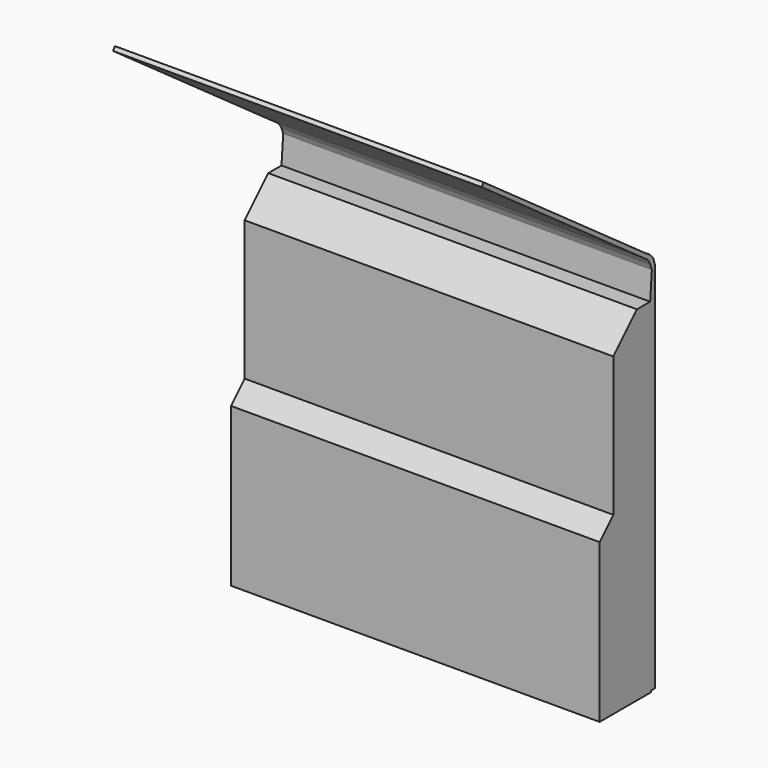
from build123d import *

# Parameters (mm, degrees)
F1_DEPTH    = 31.75
F2_T1_DEPTH = 89.6282991577
F2_T6_DEPTH = 89.6282991577
F4_DEPTH    = 31.75


# Not quite as in the source:
# - a fillet or chamfer that OpenCascade refuses, or shapes differently, is made with other operations: its cross-section is extruded or revolved along the edge and cut away or added


with BuildPart() as f1:
    # F0 (on Right) → F1 (new body, symmetric)
    with BuildSketch(Plane.YZ):
        Polygon((5.5137062445, 29.6514853835), (-2.5730628986, 29.6514853835), (-2.5730628986, 2.6955895592), (-5.5137062445, 2.6955895592), (-5.5137062445, -29.6514853835), (5.5137062445, -29.6514853835), align=None)
    extrude(amount=F1_DEPTH, both=True)

    # F2: chamfer of 5.08 on 2 edges, made by hand

    # F2_s2 → F2_t1 (cut)
    with BuildSketch(Plane.YZ.offset(-44.8141495789)):
        Polygon((2.5069371014, 29.6514853835), (-2.5730628986, 24.5714853835), (-2.5730628986, 29.6514853835), align=None)
    extrude(amount=F2_T1_DEPTH, mode=Mode.SUBTRACT)


with BuildPart() as f2_tool4:
    # F2_s5 → F2_t6 (new body)
    with BuildSketch(Plane.YZ.offset(-44.8141495789)):
        Polygon((-5.5137062445, -2.3844104408), (-0.4337062445, 2.6955895592), (-5.5137062445, 2.6955895592), align=None)
    extrude(amount=F2_T6_DEPTH)

    split(bisect_by=Plane.XZ.offset(2.5730628986), keep=Keep.TOP)


with BuildPart() as f1_1:
    add(f1.part)

    # F2_t3: cut F2_tool4
    add(f2_tool4.part, mode=Mode.SUBTRACT)

    # F3 (on Right) → F4 (join, symmetric)
    with BuildSketch(Plane.YZ):
        Polygon((5.3522153758, 29.5617226511), (5.411314778, -29.3982010335), (6.4068306237, -29.3982010335), (6.4068306237, 34.8174758255), (6.0373530723, 35.9628349543), (5.3522153758, 36.7688797414), (4.586473573, 37.2525081038), (-30.5093135685, 62.3375996947), (-30.9179358327, 61.7659087381), (4.054645617, 36.7688797414), (4.8554181121, 36.1976027489), (5.3522153758, 35.3252030909), (5.7278168388, 34.3364849687), align=None)
    extrude(amount=F4_DEPTH, both=True)


solid = f1_1.part
